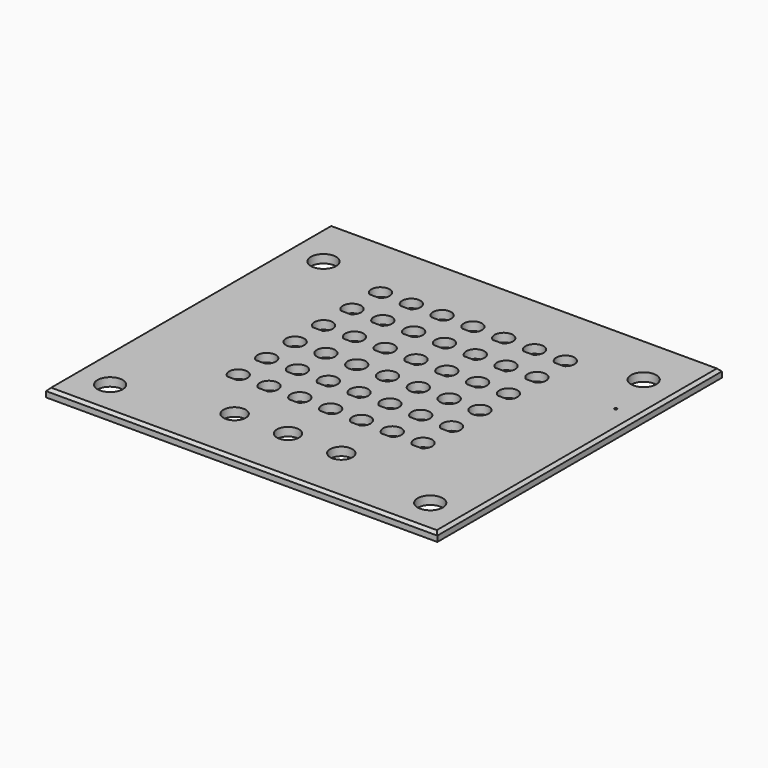
from build123d import *

# Parameters (mm, degrees)
F0_W     = 139.7
F0_H     = 127
F0_R     = 4.5
F0_R_2   = 3.97
F0_R_3   = 0.4709251225
F1_DEPTH = 3
F2_SIZE  = 1


# Not quite as in the source:
# - a feature names something its author has since deleted; it is built from what else it names


with BuildPart() as f1:
    # F0 (on Top) → F1 (new body)
    with BuildSketch(Plane.XY):
        Rectangle(F0_W, F0_H)
        with Locations((-57.15, -50.8)):
            Circle(F0_R, mode=Mode.SUBTRACT)
        with Locations((-19.05, -42.8625)):
            Circle(F0_R_2, mode=Mode.SUBTRACT)
        with BuildLine():
            ThreePointArc((-34.73, -26.5637906062), (-34.5716233646, -20.9677680267), (-29.75, -23.8125))
            ThreePointArc((-29.75, -23.8125), (-30.1552680267, -25.3841233646), (-31.27, -26.5637906062))
            ThreePointArc((-31.27, -26.5637906062), (-33, -27.0625), (-34.73, -26.5637906062))
        make_face(mode=Mode.SUBTRACT)
        with BuildLine():
            ThreePointArc((-23.73, -26.5637906062), (-23.5716233646, -20.9677680267), (-18.75, -23.8125))
            ThreePointArc((-18.75, -23.8125), (-19.1552680267, -25.3841233646), (-20.27, -26.5637906062))
            ThreePointArc((-20.27, -26.5637906062), (-22, -27.0625), (-23.73, -26.5637906062))
        make_face(mode=Mode.SUBTRACT)
        with BuildLine():
            ThreePointArc((-12.73, -26.5637906062), (-12.5716233646, -20.9677680267), (-7.75, -23.8125))
            ThreePointArc((-7.75, -23.8125), (-8.1552680267, -25.3841233646), (-9.27, -26.5637906062))
            ThreePointArc((-9.27, -26.5637906062), (-11, -27.0625), (-12.73, -26.5637906062))
        make_face(mode=Mode.SUBTRACT)
        with BuildLine():
            ThreePointArc((-34.73, -13.8637906062), (-34.5716233646, -8.2677680267), (-29.75, -11.1125))
            ThreePointArc((-29.75, -11.1125), (-30.1552680267, -12.6841233646), (-31.27, -13.8637906062))
            ThreePointArc((-31.27, -13.8637906062), (-33, -14.3625), (-34.73, -13.8637906062))
        make_face(mode=Mode.SUBTRACT)
        with BuildLine():
            ThreePointArc((-23.73, -13.8637906062), (-23.5716233646, -8.2677680267), (-18.75, -11.1125))
            ThreePointArc((-18.75, -11.1125), (-19.1552680267, -12.6841233646), (-20.27, -13.8637906062))
            ThreePointArc((-20.27, -13.8637906062), (-22, -14.3625), (-23.73, -13.8637906062))
        make_face(mode=Mode.SUBTRACT)
        with BuildLine():
            ThreePointArc((-12.73, -13.8637906062), (-12.5716233646, -8.2677680267), (-7.75, -11.1125))
            ThreePointArc((-7.75, -11.1125), (-8.1552680267, -12.6841233646), (-9.27, -13.8637906062))
            ThreePointArc((-9.27, -13.8637906062), (-11, -14.3625), (-12.73, -13.8637906062))
        make_face(mode=Mode.SUBTRACT)
        with Locations((0, -42.8625)):
            Circle(F0_R_2, mode=Mode.SUBTRACT)
        with Locations((19.05, -42.8625)):
            Circle(F0_R_2, mode=Mode.SUBTRACT)
        with Locations((57.15, -50.8)):
            Circle(F0_R, mode=Mode.SUBTRACT)
        with BuildLine():
            ThreePointArc((-1.73, -26.5637906062), (-1.5716233646, -20.9677680267), (3.25, -23.8125))
            ThreePointArc((3.25, -23.8125), (2.8447319733, -25.3841233646), (1.73, -26.5637906062))
            ThreePointArc((1.73, -26.5637906062), (0, -27.0625), (-1.73, -26.5637906062))
        make_face(mode=Mode.SUBTRACT)
        with BuildLine():
            ThreePointArc((9.27, -26.5637906062), (9.4283766354, -20.9677680267), (14.25, -23.8125))
            ThreePointArc((14.25, -23.8125), (13.8447319733, -25.3841233646), (12.73, -26.5637906062))
            ThreePointArc((12.73, -26.5637906062), (11, -27.0625), (9.27, -26.5637906062))
        make_face(mode=Mode.SUBTRACT)
        with BuildLine():
            ThreePointArc((20.27, -26.5637906062), (20.4283766354, -20.9677680267), (25.25, -23.8125))
            ThreePointArc((25.25, -23.8125), (24.8447319733, -25.3841233646), (23.73, -26.5637906062))
            ThreePointArc((23.73, -26.5637906062), (22, -27.0625), (20.27, -26.5637906062))
        make_face(mode=Mode.SUBTRACT)
        with BuildLine():
            ThreePointArc((31.27, -26.5637906062), (31.4283766354, -20.9677680267), (36.25, -23.8125))
            ThreePointArc((36.25, -23.8125), (35.8447319733, -25.3841233646), (34.73, -26.5637906062))
            ThreePointArc((34.73, -26.5637906062), (33, -27.0625), (31.27, -26.5637906062))
        make_face(mode=Mode.SUBTRACT)
        with BuildLine():
            ThreePointArc((-1.73, -13.8637906062), (-1.5716233646, -8.2677680267), (3.25, -11.1125))
            ThreePointArc((3.25, -11.1125), (2.8447319733, -12.6841233646), (1.73, -13.8637906062))
            ThreePointArc((1.73, -13.8637906062), (0, -14.3625), (-1.73, -13.8637906062))
        make_face(mode=Mode.SUBTRACT)
        with BuildLine():
            ThreePointArc((9.27, -13.8637906062), (9.4283766354, -8.2677680267), (14.25, -11.1125))
            ThreePointArc((14.25, -11.1125), (13.8447319733, -12.6841233646), (12.73, -13.8637906062))
            ThreePointArc((12.73, -13.8637906062), (11, -14.3625), (9.27, -13.8637906062))
        make_face(mode=Mode.SUBTRACT)
        with BuildLine():
            ThreePointArc((20.27, -13.8637906062), (20.4283766354, -8.2677680267), (25.25, -11.1125))
            ThreePointArc((25.25, -11.1125), (24.8447319733, -12.6841233646), (23.73, -13.8637906062))
            ThreePointArc((23.73, -13.8637906062), (22, -14.3625), (20.27, -13.8637906062))
        make_face(mode=Mode.SUBTRACT)
        with BuildLine():
            ThreePointArc((31.27, -13.8637906062), (31.4283766354, -8.2677680267), (36.25, -11.1125))
            ThreePointArc((36.25, -11.1125), (35.8447319733, -12.6841233646), (34.73, -13.8637906062))
            ThreePointArc((34.73, -13.8637906062), (33, -14.3625), (31.27, -13.8637906062))
        make_face(mode=Mode.SUBTRACT)
        with BuildLine():
            ThreePointArc((-34.73, -1.1637906062), (-34.5716233646, 4.4322319733), (-29.75, 1.5875))
            ThreePointArc((-29.75, 1.5875), (-30.1552680267, 0.0158766354), (-31.27, -1.1637906062))
            ThreePointArc((-31.27, -1.1637906062), (-33, -1.6625), (-34.73, -1.1637906062))
        make_face(mode=Mode.SUBTRACT)
        with BuildLine():
            ThreePointArc((-23.73, -1.1637906062), (-23.5716233646, 4.4322319733), (-18.75, 1.5875))
            ThreePointArc((-18.75, 1.5875), (-19.1552680267, 0.0158766354), (-20.27, -1.1637906062))
            ThreePointArc((-20.27, -1.1637906062), (-22, -1.6625), (-23.73, -1.1637906062))
        make_face(mode=Mode.SUBTRACT)
        with BuildLine():
            ThreePointArc((-34.73, 11.5362093938), (-34.5716233646, 17.1322319733), (-29.75, 14.2875))
            ThreePointArc((-29.75, 14.2875), (-30.1552680267, 12.7158766354), (-31.27, 11.5362093938))
            ThreePointArc((-31.27, 11.5362093938), (-33, 11.0375), (-34.73, 11.5362093938))
        make_face(mode=Mode.SUBTRACT)
        with BuildLine():
            ThreePointArc((-23.73, 11.5362093938), (-23.5716233646, 17.1322319733), (-18.75, 14.2875))
            ThreePointArc((-18.75, 14.2875), (-19.1552680267, 12.7158766354), (-20.27, 11.5362093938))
            ThreePointArc((-20.27, 11.5362093938), (-22, 11.0375), (-23.73, 11.5362093938))
        make_face(mode=Mode.SUBTRACT)
        with BuildLine():
            ThreePointArc((-12.73, -1.1637906062), (-12.5716233646, 4.4322319733), (-7.75, 1.5875))
            ThreePointArc((-7.75, 1.5875), (-8.1552680267, 0.0158766354), (-9.27, -1.1637906062))
            ThreePointArc((-9.27, -1.1637906062), (-11, -1.6625), (-12.73, -1.1637906062))
        make_face(mode=Mode.SUBTRACT)
        with BuildLine():
            ThreePointArc((-12.73, 11.5362093938), (-12.5716233646, 17.1322319733), (-7.75, 14.2875))
            ThreePointArc((-7.75, 14.2875), (-8.1552680267, 12.7158766354), (-9.27, 11.5362093938))
            ThreePointArc((-9.27, 11.5362093938), (-11, 11.0375), (-12.73, 11.5362093938))
        make_face(mode=Mode.SUBTRACT)
        with BuildLine():
            ThreePointArc((-34.73, 24.2362093938), (-34.5716233646, 29.8322319733), (-29.75, 26.9875))
            ThreePointArc((-29.75, 26.9875), (-30.1552680267, 25.4158766354), (-31.27, 24.2362093938))
            ThreePointArc((-31.27, 24.2362093938), (-33, 23.7375), (-34.73, 24.2362093938))
        make_face(mode=Mode.SUBTRACT)
        with BuildLine():
            ThreePointArc((-23.73, 24.2362093938), (-23.5716233646, 29.8322319733), (-18.75, 26.9875))
            ThreePointArc((-18.75, 26.9875), (-19.1552680267, 25.4158766354), (-20.27, 24.2362093938))
            ThreePointArc((-20.27, 24.2362093938), (-22, 23.7375), (-23.73, 24.2362093938))
        make_face(mode=Mode.SUBTRACT)
        with BuildLine():
            ThreePointArc((-12.73, 24.2362093938), (-12.5716233646, 29.8322319733), (-7.75, 26.9875))
            ThreePointArc((-7.75, 26.9875), (-8.1552680267, 25.4158766354), (-9.27, 24.2362093938))
            ThreePointArc((-9.27, 24.2362093938), (-11, 23.7375), (-12.73, 24.2362093938))
        make_face(mode=Mode.SUBTRACT)
        with Locations((-57.157959789, 44.45)):
            Circle(F0_R, mode=Mode.SUBTRACT)
        with BuildLine():
            ThreePointArc((-34.73, 36.9362093938), (-34.5716233646, 42.5322319733), (-29.75, 39.6875))
            ThreePointArc((-29.75, 39.6875), (-30.1552680267, 38.1158766354), (-31.27, 36.9362093938))
            ThreePointArc((-31.27, 36.9362093938), (-33, 36.4375), (-34.73, 36.9362093938))
        make_face(mode=Mode.SUBTRACT)
        with BuildLine():
            ThreePointArc((-23.73, 36.9362093938), (-23.5716233646, 42.5322319733), (-18.75, 39.6875))
            ThreePointArc((-18.75, 39.6875), (-19.1552680267, 38.1158766354), (-20.27, 36.9362093938))
            ThreePointArc((-20.27, 36.9362093938), (-22, 36.4375), (-23.73, 36.9362093938))
        make_face(mode=Mode.SUBTRACT)
        with BuildLine():
            ThreePointArc((-12.73, 36.9362093938), (-12.5716233646, 42.5322319733), (-7.75, 39.6875))
            ThreePointArc((-7.75, 39.6875), (-8.1552680267, 38.1158766354), (-9.27, 36.9362093938))
            ThreePointArc((-9.27, 36.9362093938), (-11, 36.4375), (-12.73, 36.9362093938))
        make_face(mode=Mode.SUBTRACT)
        with BuildLine():
            ThreePointArc((-1.73, -1.1637906062), (-1.5716233646, 4.4322319733), (3.25, 1.5875))
            ThreePointArc((3.25, 1.5875), (2.8447319733, 0.0158766354), (1.73, -1.1637906062))
            ThreePointArc((1.73, -1.1637906062), (0, -1.6625), (-1.73, -1.1637906062))
        make_face(mode=Mode.SUBTRACT)
        with BuildLine():
            ThreePointArc((9.27, -1.1637906062), (9.4283766354, 4.4322319733), (14.25, 1.5875))
            ThreePointArc((14.25, 1.5875), (13.8447319733, 0.0158766354), (12.73, -1.1637906062))
            ThreePointArc((12.73, -1.1637906062), (11, -1.6625), (9.27, -1.1637906062))
        make_face(mode=Mode.SUBTRACT)
        with BuildLine():
            ThreePointArc((-1.73, 11.5362093938), (-1.5716233646, 17.1322319733), (3.25, 14.2875))
            ThreePointArc((3.25, 14.2875), (2.8447319733, 12.7158766354), (1.73, 11.5362093938))
            ThreePointArc((1.73, 11.5362093938), (0, 11.0375), (-1.73, 11.5362093938))
        make_face(mode=Mode.SUBTRACT)
        with BuildLine():
            ThreePointArc((9.27, 11.5362093938), (9.4283766354, 17.1322319733), (14.25, 14.2875))
            ThreePointArc((14.25, 14.2875), (13.8447319733, 12.7158766354), (12.73, 11.5362093938))
            ThreePointArc((12.73, 11.5362093938), (11, 11.0375), (9.27, 11.5362093938))
        make_face(mode=Mode.SUBTRACT)
        with BuildLine():
            ThreePointArc((20.27, -1.1637906062), (20.4283766354, 4.4322319733), (25.25, 1.5875))
            ThreePointArc((25.25, 1.5875), (24.8447319733, 0.0158766354), (23.73, -1.1637906062))
            ThreePointArc((23.73, -1.1637906062), (22, -1.6625), (20.27, -1.1637906062))
        make_face(mode=Mode.SUBTRACT)
        with BuildLine():
            ThreePointArc((31.27, -1.1637906062), (31.4283766354, 4.4322319733), (36.25, 1.5875))
            ThreePointArc((36.25, 1.5875), (35.8447319733, 0.0158766354), (34.73, -1.1637906062))
            ThreePointArc((34.73, -1.1637906062), (33, -1.6625), (31.27, -1.1637906062))
        make_face(mode=Mode.SUBTRACT)
        with BuildLine():
            ThreePointArc((20.27, 11.5362093938), (20.4283766354, 17.1322319733), (25.25, 14.2875))
            ThreePointArc((25.25, 14.2875), (24.8447319733, 12.7158766354), (23.73, 11.5362093938))
            ThreePointArc((23.73, 11.5362093938), (22, 11.0375), (20.27, 11.5362093938))
        make_face(mode=Mode.SUBTRACT)
        with BuildLine():
            ThreePointArc((31.27, 11.5362093938), (31.4283766354, 17.1322319733), (36.25, 14.2875))
            ThreePointArc((36.25, 14.2875), (35.8447319733, 12.7158766354), (34.73, 11.5362093938))
            ThreePointArc((34.73, 11.5362093938), (33, 11.0375), (31.27, 11.5362093938))
        make_face(mode=Mode.SUBTRACT)
        with BuildLine():
            ThreePointArc((-1.73, 24.2362093938), (-1.5716233646, 29.8322319733), (3.25, 26.9875))
            ThreePointArc((3.25, 26.9875), (2.8447319733, 25.4158766354), (1.73, 24.2362093938))
            ThreePointArc((1.73, 24.2362093938), (0, 23.7375), (-1.73, 24.2362093938))
        make_face(mode=Mode.SUBTRACT)
        with BuildLine():
            ThreePointArc((9.27, 24.2362093938), (9.4283766354, 29.8322319733), (14.25, 26.9875))
            ThreePointArc((14.25, 26.9875), (13.8447319733, 25.4158766354), (12.73, 24.2362093938))
            ThreePointArc((12.73, 24.2362093938), (11, 23.7375), (9.27, 24.2362093938))
        make_face(mode=Mode.SUBTRACT)
        with BuildLine():
            ThreePointArc((20.27, 24.2362093938), (20.4283766354, 29.8322319733), (25.25, 26.9875))
            ThreePointArc((25.25, 26.9875), (24.8447319733, 25.4158766354), (23.73, 24.2362093938))
            ThreePointArc((23.73, 24.2362093938), (22, 23.7375), (20.27, 24.2362093938))
        make_face(mode=Mode.SUBTRACT)
        with BuildLine():
            ThreePointArc((31.27, 24.2362093938), (31.4283766354, 29.8322319733), (36.25, 26.9875))
            ThreePointArc((36.25, 26.9875), (35.8447319733, 25.4158766354), (34.73, 24.2362093938))
            ThreePointArc((34.73, 24.2362093938), (33, 23.7375), (31.27, 24.2362093938))
        make_face(mode=Mode.SUBTRACT)
        with Locations((61.9865506887, 25.8642937988)):
            Circle(F0_R_3, mode=Mode.SUBTRACT)
        with BuildLine():
            ThreePointArc((-1.73, 36.9362093938), (-1.5716233646, 42.5322319733), (3.25, 39.6875))
            ThreePointArc((3.25, 39.6875), (2.8447319733, 38.1158766354), (1.73, 36.9362093938))
            ThreePointArc((1.73, 36.9362093938), (0, 36.4375), (-1.73, 36.9362093938))
        make_face(mode=Mode.SUBTRACT)
        with BuildLine():
            ThreePointArc((9.27, 36.9362093938), (9.4283766354, 42.5322319733), (14.25, 39.6875))
            ThreePointArc((14.25, 39.6875), (13.8447319733, 38.1158766354), (12.73, 36.9362093938))
            ThreePointArc((12.73, 36.9362093938), (11, 36.4375), (9.27, 36.9362093938))
        make_face(mode=Mode.SUBTRACT)
        with BuildLine():
            ThreePointArc((20.27, 36.9362093938), (20.4283766354, 42.5322319733), (25.25, 39.6875))
            ThreePointArc((25.25, 39.6875), (24.8447319733, 38.1158766354), (23.73, 36.9362093938))
            ThreePointArc((23.73, 36.9362093938), (22, 36.4375), (20.27, 36.9362093938))
        make_face(mode=Mode.SUBTRACT)
        with BuildLine():
            ThreePointArc((31.27, 36.9362093938), (31.4283766354, 42.5322319733), (36.25, 39.6875))
            ThreePointArc((36.25, 39.6875), (35.8447319733, 38.1158766354), (34.73, 36.9362093938))
            ThreePointArc((34.73, 36.9362093938), (33, 36.4375), (31.27, 36.9362093938))
        make_face(mode=Mode.SUBTRACT)
        with Locations((57.15, 44.45)):
            Circle(F0_R, mode=Mode.SUBTRACT)
        with BuildLine():
            Line((-31.27, 36.9362093938), (-34.73, 36.9362093938))
            ThreePointArc((-34.73, 36.9362093938), (-33, 36.4375), (-31.27, 36.9362093938))
        make_face()
        with BuildLine():
            Line((-20.27, 36.9362093938), (-23.73, 36.9362093938))
            ThreePointArc((-23.73, 36.9362093938), (-22, 36.4375), (-20.27, 36.9362093938))
        make_face()
        with BuildLine():
            Line((-9.27, 36.9362093938), (-12.73, 36.9362093938))
            ThreePointArc((-12.73, 36.9362093938), (-11, 36.4375), (-9.27, 36.9362093938))
        make_face()
        with BuildLine():
            Line((1.73, 36.9362093938), (-1.73, 36.9362093938))
            ThreePointArc((-1.73, 36.9362093938), (0, 36.4375), (1.73, 36.9362093938))
        make_face()
        with BuildLine():
            Line((1.73, 24.2362093938), (-1.73, 24.2362093938))
            ThreePointArc((-1.73, 24.2362093938), (0, 23.7375), (1.73, 24.2362093938))
        make_face()
        with BuildLine():
            Line((-9.27, 24.2362093938), (-12.73, 24.2362093938))
            ThreePointArc((-12.73, 24.2362093938), (-11, 23.7375), (-9.27, 24.2362093938))
        make_face()
        with BuildLine():
            Line((-20.27, 24.2362093938), (-23.73, 24.2362093938))
            ThreePointArc((-23.73, 24.2362093938), (-22, 23.7375), (-20.27, 24.2362093938))
        make_face()
        with BuildLine():
            Line((-31.27, 24.2362093938), (-34.73, 24.2362093938))
            ThreePointArc((-34.73, 24.2362093938), (-33, 23.7375), (-31.27, 24.2362093938))
        make_face()
        with BuildLine():
            Line((12.73, 36.9362093938), (9.27, 36.9362093938))
            ThreePointArc((9.27, 36.9362093938), (11, 36.4375), (12.73, 36.9362093938))
        make_face()
        with BuildLine():
            Line((23.73, 36.9362093938), (20.27, 36.9362093938))
            ThreePointArc((20.27, 36.9362093938), (22, 36.4375), (23.73, 36.9362093938))
        make_face()
        with BuildLine():
            Line((34.73, 36.9362093938), (31.27, 36.9362093938))
            ThreePointArc((31.27, 36.9362093938), (33, 36.4375), (34.73, 36.9362093938))
        make_face()
        with BuildLine():
            Line((34.73, 24.2362093938), (31.27, 24.2362093938))
            ThreePointArc((31.27, 24.2362093938), (33, 23.7375), (34.73, 24.2362093938))
        make_face()
        with BuildLine():
            Line((23.73, 24.2362093938), (20.27, 24.2362093938))
            ThreePointArc((20.27, 24.2362093938), (22, 23.7375), (23.73, 24.2362093938))
        make_face()
        with BuildLine():
            Line((12.73, 24.2362093938), (9.27, 24.2362093938))
            ThreePointArc((9.27, 24.2362093938), (11, 23.7375), (12.73, 24.2362093938))
        make_face()
        with BuildLine():
            Line((34.73, 11.5362093938), (31.27, 11.5362093938))
            ThreePointArc((31.27, 11.5362093938), (33, 11.0375), (34.73, 11.5362093938))
        make_face()
        with BuildLine():
            Line((12.73, 11.5362093938), (9.27, 11.5362093938))
            ThreePointArc((9.27, 11.5362093938), (11, 11.0375), (12.73, 11.5362093938))
        make_face()
        with BuildLine():
            Line((23.73, 11.5362093938), (20.27, 11.5362093938))
            ThreePointArc((20.27, 11.5362093938), (22, 11.0375), (23.73, 11.5362093938))
        make_face()
        with BuildLine():
            Line((1.73, 11.5362093938), (-1.73, 11.5362093938))
            ThreePointArc((-1.73, 11.5362093938), (0, 11.0375), (1.73, 11.5362093938))
        make_face()
        with BuildLine():
            Line((-9.27, 11.5362093938), (-12.73, 11.5362093938))
            ThreePointArc((-12.73, 11.5362093938), (-11, 11.0375), (-9.27, 11.5362093938))
        make_face()
        with BuildLine():
            Line((-20.27, 11.5362093938), (-23.73, 11.5362093938))
            ThreePointArc((-23.73, 11.5362093938), (-22, 11.0375), (-20.27, 11.5362093938))
        make_face()
        with BuildLine():
            Line((-31.27, 11.5362093938), (-34.73, 11.5362093938))
            ThreePointArc((-34.73, 11.5362093938), (-33, 11.0375), (-31.27, 11.5362093938))
        make_face()
        with BuildLine():
            Line((-31.27, -13.8637906062), (-34.73, -13.8637906062))
            ThreePointArc((-34.73, -13.8637906062), (-33, -14.3625), (-31.27, -13.8637906062))
        make_face()
        with BuildLine():
            Line((-31.27, -26.5637906062), (-34.73, -26.5637906062))
            ThreePointArc((-34.73, -26.5637906062), (-33, -27.0625), (-31.27, -26.5637906062))
        make_face()
        with BuildLine():
            Line((-20.27, -26.5637906062), (-23.73, -26.5637906062))
            ThreePointArc((-23.73, -26.5637906062), (-22, -27.0625), (-20.27, -26.5637906062))
        make_face()
        with BuildLine():
            Line((-20.27, -13.8637906062), (-23.73, -13.8637906062))
            ThreePointArc((-23.73, -13.8637906062), (-22, -14.3625), (-20.27, -13.8637906062))
        make_face()
        with BuildLine():
            Line((-9.27, -13.8637906062), (-12.73, -13.8637906062))
            ThreePointArc((-12.73, -13.8637906062), (-11, -14.3625), (-9.27, -13.8637906062))
        make_face()
        with BuildLine():
            Line((-9.27, -26.5637906062), (-12.73, -26.5637906062))
            ThreePointArc((-12.73, -26.5637906062), (-11, -27.0625), (-9.27, -26.5637906062))
        make_face()
        with BuildLine():
            Line((1.73, -26.5637906062), (-1.73, -26.5637906062))
            ThreePointArc((-1.73, -26.5637906062), (0, -27.0625), (1.73, -26.5637906062))
        make_face()
        with BuildLine():
            Line((1.73, -13.8637906062), (-1.73, -13.8637906062))
            ThreePointArc((-1.73, -13.8637906062), (0, -14.3625), (1.73, -13.8637906062))
        make_face()
        with BuildLine():
            Line((12.73, -13.8637906062), (9.27, -13.8637906062))
            ThreePointArc((9.27, -13.8637906062), (11, -14.3625), (12.73, -13.8637906062))
        make_face()
        with BuildLine():
            Line((23.73, -13.8637906062), (20.27, -13.8637906062))
            ThreePointArc((20.27, -13.8637906062), (22, -14.3625), (23.73, -13.8637906062))
        make_face()
        with BuildLine():
            Line((34.73, -13.8637906062), (31.27, -13.8637906062))
            ThreePointArc((31.27, -13.8637906062), (33, -14.3625), (34.73, -13.8637906062))
        make_face()
        with BuildLine():
            Line((34.73, -26.5637906062), (31.27, -26.5637906062))
            ThreePointArc((31.27, -26.5637906062), (33, -27.0625), (34.73, -26.5637906062))
        make_face()
        with BuildLine():
            Line((23.73, -26.5637906062), (20.27, -26.5637906062))
            ThreePointArc((20.27, -26.5637906062), (22, -27.0625), (23.73, -26.5637906062))
        make_face()
        with BuildLine():
            Line((12.73, -26.5637906062), (9.27, -26.5637906062))
            ThreePointArc((9.27, -26.5637906062), (11, -27.0625), (12.73, -26.5637906062))
        make_face()
    extrude(amount=F1_DEPTH)

    # F2
    f2_edges = [f1.edges().sort_by_distance(p)[0] for p in [
        (-69.85, 0, 3),
        (0, -63.5, 3),
        (69.85, 0, 3),
        (0, 63.5, 3),
    ]]
    chamfer(f2_edges, length=F2_SIZE)


solid = f1.part
